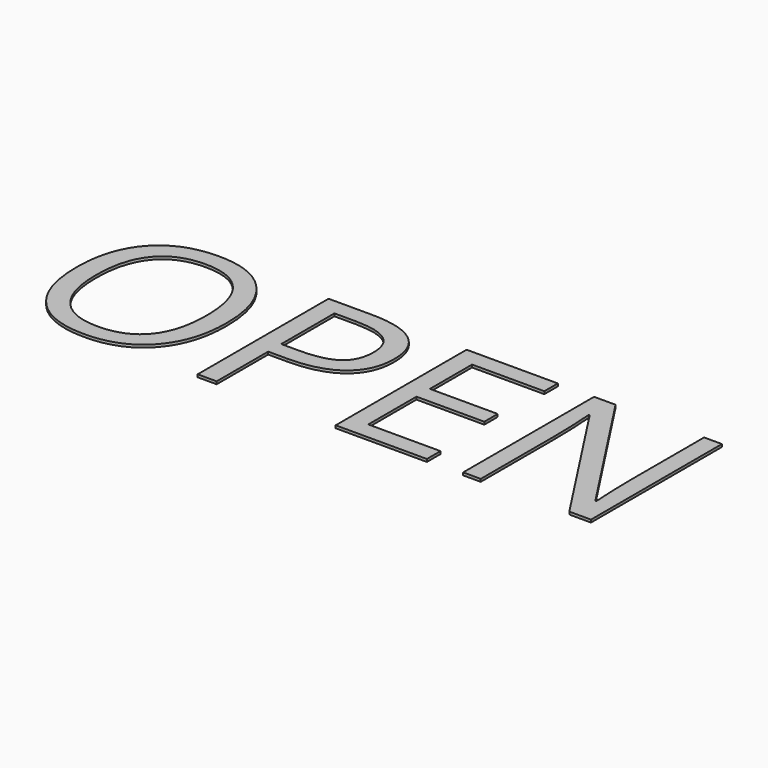
from build123d import *

# Parameters (mm, degrees)
F0_TEXT_SIZE = 34.6534678506
F1_DEPTH     = 0.4


# Not quite as in the source:
# - Text() gives the source's letters only with a copy of the font that has no kerning and outlines rounded to 1/6400 em; it was checked with that copy


with BuildPart() as f1:
    # F0 (on Top) → F1 (new body)
    with BuildSketch(Plane.XY):
        with Locations((-46.0024774075, -12.3193077743)):
            Text('OPEN', F0_TEXT_SIZE, font='Open Sans', text_align=(TextAlign.LEFT, TextAlign.BOTTOM))
    extrude(amount=F1_DEPTH)


solid = f1.part
